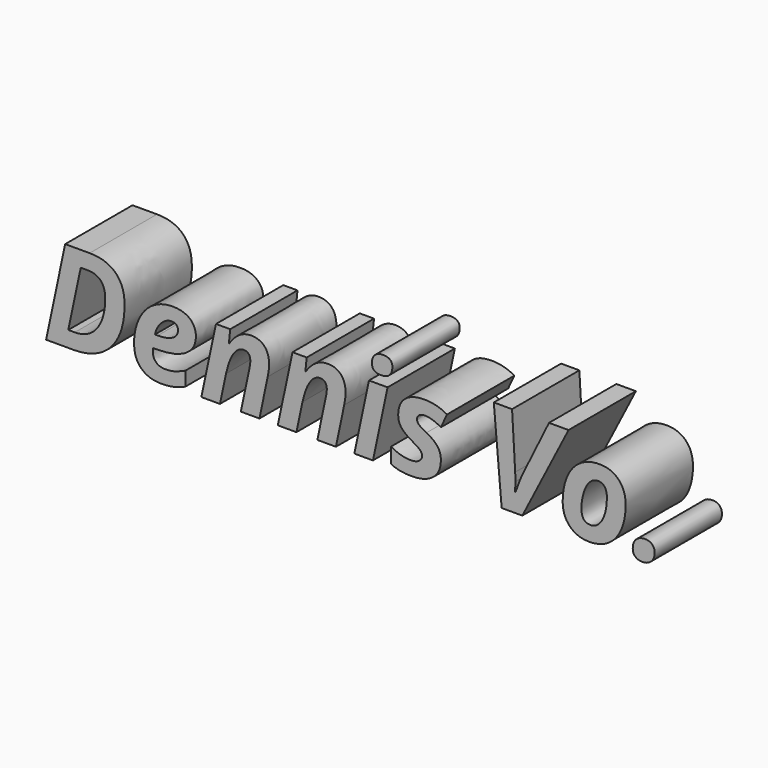
from build123d import *

# Parameters (mm, degrees)
F0_TEXT_SIZE = 38.2280559279
F1_DEPTH     = 25.4


# Not quite as in the source:
# - Text() gives the source's letters only with a copy of the font that has no kerning and outlines rounded to 1/6400 em; it was checked with that copy


with BuildPart() as f1:
    # F0 (on Front) → F1 (new body)
    with BuildSketch(Plane.XZ):
        with Locations((-91.873886995, -8.4470817819)):
            Text('Dennis Vo.', F0_TEXT_SIZE, font='Open Sans', font_style=FontStyle.BOLDITALIC, text_align=(TextAlign.LEFT, TextAlign.BOTTOM))
    extrude(amount=F1_DEPTH)


solid = f1.part
